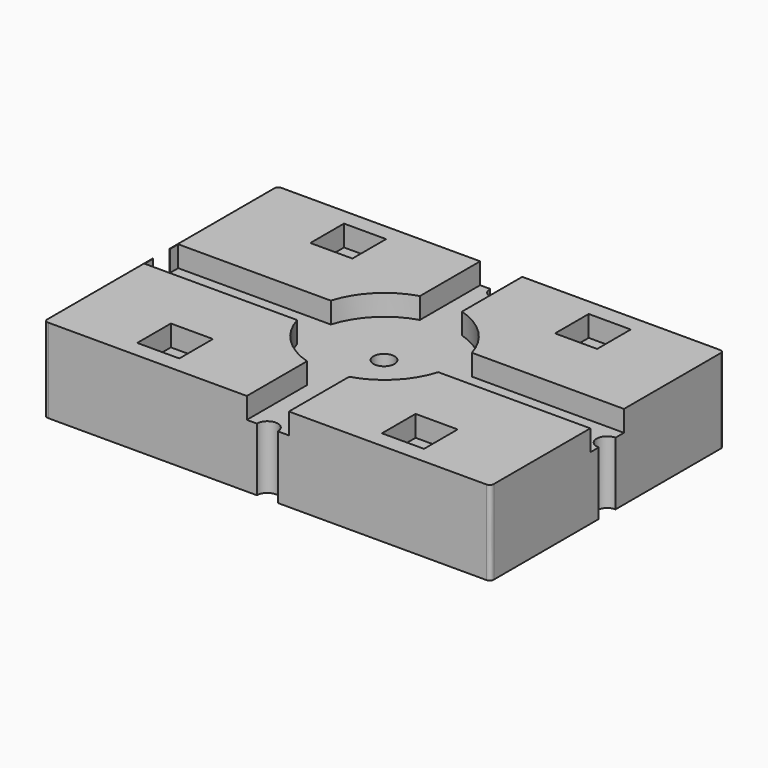
from build123d import *

# Parameters (mm, degrees)
F1_DEPTH    = 20
F3_DEPTH    = 5
F4_W        = 10
F4_H        = 10
F5_DEPTH    = 5
F6_D        = 5
F7_D        = 5
F8_T1_DEPTH = 25


# Not quite as in the source:
# - a fillet or chamfer that OpenCascade refuses, or shapes differently, is made with other operations: its cross-section is extruded or revolved along the edge and cut away or added


with BuildPart() as f1:
    # F0 (on Top) → F1 (new body)
    with BuildSketch(Plane.XY):
        with BuildLine():
            Line((16.7705098646, 4.9999998882), (53.0298836529, 4.9999998882))
            Line((53.0298836529, 4.9999998882), (53.0298836529, 34.6554927528))
            Line((53.0298836529, 34.6554927528), (5, 34.6554927528))
            Line((5, 34.6554927528), (5, 16.7705098312))
            ThreePointArc((5, 16.7705098312), (12.374368712, 12.3743686295), (16.7705098646, 4.9999998882))
        make_face()
        with BuildLine():
            Line((5, 16.7705098312), (5, 34.6554927528))
            Line((5, 34.6554927528), (-5, 34.6554927528))
            Line((-5, 34.6554927528), (-5, 16.7705098312))
            ThreePointArc((-5, 16.7705098312), (0, 17.5), (5, 16.7705098312))
        make_face()
        with BuildLine():
            Line((-53.0298836529, 34.6554927528), (-53.0298836529, 4.9999998882))
            Line((-53.0298836529, 4.9999998882), (-16.7705098646, 4.9999998882))
            ThreePointArc((-16.7705098646, 4.9999998882), (-12.374368712, 12.3743686295), (-5, 16.7705098312))
            Line((-5, 16.7705098312), (-5, 34.6554927528))
            Line((-5, 34.6554927528), (-53.0298836529, 34.6554927528))
        make_face()
        with BuildLine():
            Line((-53.0298836529, -34.6554927528), (-5, -34.6554927528))
            Line((-5, -34.6554927528), (-5, -16.7705098312))
            ThreePointArc((-5, -16.7705098312), (-12.374368712, -12.3743686295), (-16.7705098646, -4.9999998882))
            Line((-16.7705098646, -4.9999998882), (-53.0298836529, -4.9999998882))
            Line((-53.0298836529, -4.9999998882), (-53.0298836529, -34.6554927528))
        make_face()
        with BuildLine():
            Line((5, -34.6554927528), (53.0298836529, -34.6554927528))
            Line((53.0298836529, -34.6554927528), (53.0298836529, -4.9999998882))
            Line((53.0298836529, -4.9999998882), (16.7705098646, -4.9999998882))
            ThreePointArc((16.7705098646, -4.9999998882), (12.374368712, -12.3743686295), (5, -16.7705098312))
            Line((5, -16.7705098312), (5, -34.6554927528))
        make_face()
        with BuildLine():
            Line((16.7705098646, -4.9999998882), (53.0298836529, -4.9999998882))
            Line((53.0298836529, -4.9999998882), (53.0298836529, 4.9999998882))
            Line((53.0298836529, 4.9999998882), (16.7705098646, 4.9999998882))
            ThreePointArc((16.7705098646, 4.9999998882), (17.3166671538, 2.5264676299), (17.5, 0))
            ThreePointArc((17.5, 0), (17.3166671538, -2.5264676299), (16.7705098646, -4.9999998882))
        make_face()
        with BuildLine():
            ThreePointArc((-5, -16.7705098312), (0, -17.5), (5, -16.7705098312))
            ThreePointArc((5, -16.7705098312), (12.374368712, -12.3743686295), (16.7705098646, -4.9999998882))
            ThreePointArc((16.7705098646, -4.9999998882), (17.3166671538, -2.5264676299), (17.5, 0))
            ThreePointArc((17.5, 0), (17.3166671538, 2.5264676299), (16.7705098646, 4.9999998882))
            ThreePointArc((16.7705098646, 4.9999998882), (12.374368712, 12.3743686295), (5, 16.7705098312))
            ThreePointArc((5, 16.7705098312), (0, 17.5), (-5, 16.7705098312))
            ThreePointArc((-5, 16.7705098312), (-12.374368712, 12.3743686295), (-16.7705098646, 4.9999998882))
            ThreePointArc((-16.7705098646, 4.9999998882), (-17.5, 0), (-16.7705098646, -4.9999998882))
            ThreePointArc((-16.7705098646, -4.9999998882), (-12.374368712, -12.3743686295), (-5, -16.7705098312))
        make_face()
        with BuildLine():
            Line((-53.0298836529, 4.9999998882), (-53.0298836529, -4.9999998882))
            Line((-53.0298836529, -4.9999998882), (-16.7705098646, -4.9999998882))
            ThreePointArc((-16.7705098646, -4.9999998882), (-17.5, 0), (-16.7705098646, 4.9999998882))
            Line((-16.7705098646, 4.9999998882), (-53.0298836529, 4.9999998882))
        make_face()
        with BuildLine():
            Line((-5, -34.6554927528), (5, -34.6554927528))
            Line((5, -34.6554927528), (5, -16.7705098312))
            ThreePointArc((5, -16.7705098312), (0, -17.5), (-5, -16.7705098312))
            Line((-5, -16.7705098312), (-5, -34.6554927528))
        make_face()
    extrude(amount=F1_DEPTH)

    # F2 (on face) → F3 (cut)
    with BuildSketch(Plane.XY.offset(20)):
        with BuildLine():
            Line((-52.9048836529, 4.9999998882), (-52.9048836529, -4.9999998882))
            Line((-52.9048836529, -4.9999998882), (-16.6455098646, -4.9999998882))
            ThreePointArc((-16.6455098646, -4.9999998882), (-17.375, 0), (-16.6455098646, 4.9999998882))
            Line((-16.6455098646, 4.9999998882), (-52.9048836529, 4.9999998882))
        make_face()
        with BuildLine():
            ThreePointArc((-4.875, 16.7705098312), (0.125, 17.5), (5.125, 16.7705098312))
            Line((5.125, 16.7705098312), (5.125, 34.6554927528))
            Line((5.125, 34.6554927528), (-4.875, 34.6554927528))
            Line((-4.875, 34.6554927528), (-4.875, 16.7705098312))
        make_face()
        with BuildLine():
            ThreePointArc((-4.875, -16.7705098312), (0.125, -17.5), (5.125, -16.7705098312))
            ThreePointArc((5.125, -16.7705098312), (12.499368712, -12.3743686295), (16.8955098646, -4.9999998882))
            ThreePointArc((16.8955098646, -4.9999998882), (17.4416671538, -2.5264676299), (17.625, 0))
            ThreePointArc((17.625, 0), (17.4416671538, 2.5264676299), (16.8955098646, 4.9999998882))
            ThreePointArc((16.8955098646, 4.9999998882), (12.499368712, 12.3743686295), (5.125, 16.7705098312))
            ThreePointArc((5.125, 16.7705098312), (0.125, 17.5), (-4.875, 16.7705098312))
            ThreePointArc((-4.875, 16.7705098312), (-12.249368712, 12.3743686295), (-16.6455098646, 4.9999998882))
            ThreePointArc((-16.6455098646, 4.9999998882), (-17.375, 0), (-16.6455098646, -4.9999998882))
            ThreePointArc((-16.6455098646, -4.9999998882), (-12.249368712, -12.3743686295), (-4.875, -16.7705098312))
        make_face()
        with BuildLine():
            Line((16.8955098646, -4.9999998882), (53.0298836529, -4.9999998882))
            Line((53.0298836529, -4.9999998882), (53.0298836529, 4.9999998882))
            Line((53.0298836529, 4.9999998882), (16.8955098646, 4.9999998882))
            ThreePointArc((16.8955098646, 4.9999998882), (17.4416671538, 2.5264676299), (17.625, 0))
            ThreePointArc((17.625, 0), (17.4416671538, -2.5264676299), (16.8955098646, -4.9999998882))
        make_face()
        with BuildLine():
            Line((-4.875, -34.6554927528), (5.125, -34.6554927528))
            Line((5.125, -34.6554927528), (5.125, -16.7705098312))
            ThreePointArc((5.125, -16.7705098312), (0.125, -17.5), (-4.875, -16.7705098312))
            Line((-4.875, -16.7705098312), (-4.875, -34.6554927528))
        make_face()
    extrude(amount=-F3_DEPTH, mode=Mode.SUBTRACT)

    # F4 (on face) → F5 (cut)
    with BuildSketch(Plane.XY.offset(20)):
        with Locations((-29.0774418265, 25.713001292)):
            Rectangle(F4_W, F4_H)
        with Locations((29.0774418265, 25.713001292)):
            Rectangle(F4_W, F4_H)
        with Locations((29.0774418265, -25.713001292)):
            Rectangle(F4_W, F4_H)
        with Locations((-29.0774418265, -25.713001292)):
            Rectangle(F4_W, F4_H)
    extrude(amount=-F5_DEPTH, mode=Mode.SUBTRACT)

    # F6 (through all)
    with Locations(Plane(origin=(0, 0, 0), x_dir=(1, 0, 0), z_dir=(0, 0, -1))):
        with Locations((0, 34.6554927528), (0, -34.6554927528), (-53.0298836529, 0), (0, 0)):
            Hole(F6_D / 2)

    # F7 (through all)
    with Locations(Plane(origin=(0, 0, 0), x_dir=(1, 0, 0), z_dir=(0, 0, -1))):
        with Locations((53.0298836529, 0)):
            Hole(F7_D / 2)

    # F8: fillet of radius 1 on 4 edges, made by hand

    # F8_s2 → F8_t1 (cut)
    with BuildSketch(Plane.XY.offset(-2.5)):
        with BuildLine():
            add(Edge.make_bspline(
                [(52.0298836529, -34.6554927528), (53.0298836529, -34.6554927528), (53.0298836529, -33.6554927528)],
                knots=[0, 0, 0, 1, 1, 1], degree=2, weights=[1, 1, 1]))
            Line((53.0298836529, -33.6554927528), (53.0298836529, -34.6554927528))
            Line((53.0298836529, -34.6554927528), (52.0298836529, -34.6554927528))
        make_face()
        with BuildLine():
            add(Edge.make_bspline(
                [(52.0298836529, 34.6554927528), (53.0298836529, 34.6554927528), (53.0298836529, 33.6554927528)],
                knots=[0, 0, 0, 1, 1, 1], degree=2, weights=[1, 1, 1]))
            Line((53.0298836529, 33.6554927528), (53.0298836529, 34.6554927528))
            Line((53.0298836529, 34.6554927528), (52.0298836529, 34.6554927528))
        make_face()
        with BuildLine():
            add(Edge.make_bspline(
                [(-52.0298836529, -34.6554927528), (-53.0298836529, -34.6554927528), (-53.0298836529, -33.6554927528)],
                knots=[0, 0, 0, 1, 1, 1], degree=2, weights=[1, 1, 1]))
            Line((-53.0298836529, -33.6554927528), (-53.0298836529, -34.6554927528))
            Line((-53.0298836529, -34.6554927528), (-52.0298836529, -34.6554927528))
        make_face()
        with BuildLine():
            add(Edge.make_bspline(
                [(-53.0298836529, 33.6554927528), (-53.0298836529, 34.6554927528), (-52.0298836529, 34.6554927528)],
                knots=[0, 0, 0, 1, 1, 1], degree=2, weights=[1, 1, 1]))
            Line((-52.0298836529, 34.6554927528), (-53.0298836529, 34.6554927528))
            Line((-53.0298836529, 34.6554927528), (-53.0298836529, 33.6554927528))
        make_face()
    extrude(amount=F8_T1_DEPTH, mode=Mode.SUBTRACT)


solid = f1.part
